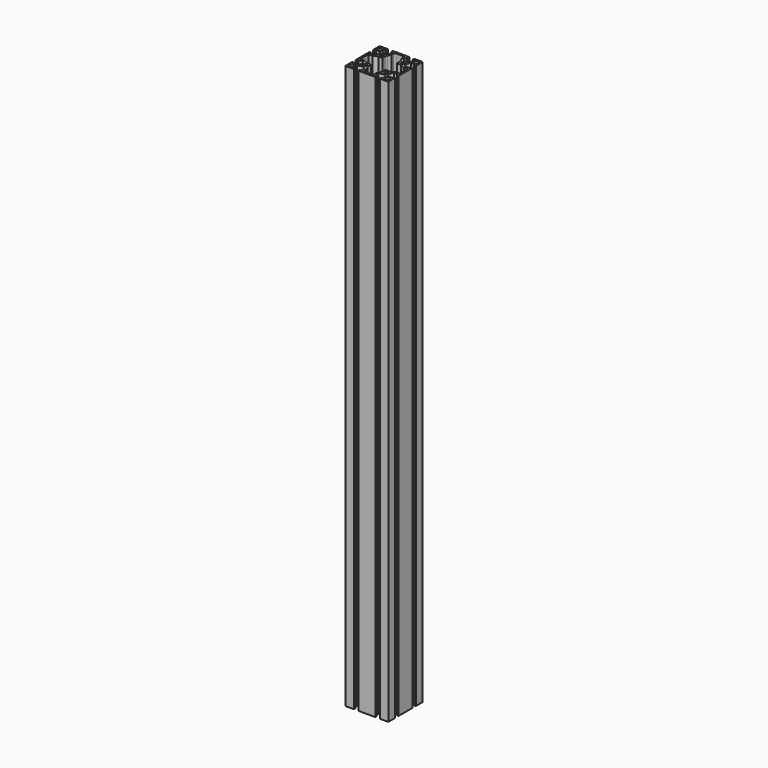
from build123d import *

# Parameters (mm, degrees)
F0_R     = 3
F0_R_2   = 2.5
F1_DEPTH = 787
F2_R     = 2
F3_R     = 7


# Not quite as in the source:
# - a feature names something its author has since deleted; it is built from what else it names


with BuildPart() as f1:
    # F0 (on Top) → F1 (new body)
    with BuildSketch(Plane.XY):
        with BuildLine():
            Line((18.15, -30), (30, -30))
            Line((30, -30), (30, -18.15))
            Line((30, -18.15), (27.5, -18.15))
            Line((27.5, -18.15), (27.5, -20.15))
            Line((27.5, -20.15), (21.5477069044, -20.15))
            ThreePointArc((21.5477069044, -20.15), (19.5, -15), (21.5477069044, -9.85))
            Line((21.5477069044, -9.85), (27.5, -9.85))
            Line((27.5, -9.85), (27.5, -11.85))
            Line((27.5, -11.85), (30, -11.85))
            Line((30, -11.85), (30, 11.85))
            Line((30, 11.85), (27.5, 11.85))
            Line((27.5, 11.85), (27.5, 9.85))
            Line((27.5, 9.85), (21.5477069044, 9.85))
            ThreePointArc((21.5477069044, 9.85), (19.5, 15), (21.5477069044, 20.15))
            Line((21.5477069044, 20.15), (27.5, 20.15))
            Line((27.5, 20.15), (27.5, 18.15))
            Line((27.5, 18.15), (30, 18.15))
            Line((30, 18.15), (30, 30))
            Line((30, 30), (18.15, 30))
            Line((18.15, 30), (18.15, 27.5))
            Line((18.15, 27.5), (20.15, 27.5))
            Line((20.15, 27.5), (20.15, 21.5477069044))
            ThreePointArc((20.15, 21.5477069044), (15, 19.5), (9.85, 21.5477069044))
            Line((9.85, 21.5477069044), (9.85, 27.5))
            Line((9.85, 27.5), (11.85, 27.5))
            Line((11.85, 27.5), (11.85, 30))
            Line((11.85, 30), (-11.85, 30))
            Line((-11.85, 30), (-11.85, 27.5))
            Line((-11.85, 27.5), (-9.85, 27.5))
            Line((-9.85, 27.5), (-9.85, 21.5477069044))
            ThreePointArc((-9.85, 21.5477069044), (-15, 19.5), (-20.15, 21.5477069044))
            Line((-20.15, 21.5477069044), (-20.15, 27.5))
            Line((-20.15, 27.5), (-18.15, 27.5))
            Line((-18.15, 27.5), (-18.15, 30))
            Line((-18.15, 30), (-30, 30))
            Line((-30, 30), (-30, 18.15))
            Line((-30, 18.15), (-27.5, 18.15))
            Line((-27.5, 18.15), (-27.5, 20.15))
            Line((-27.5, 20.15), (-21.5477069044, 20.15))
            ThreePointArc((-21.5477069044, 20.15), (-19.5, 15), (-21.5477069044, 9.85))
            Line((-21.5477069044, 9.85), (-27.5, 9.85))
            Line((-27.5, 9.85), (-27.5, 11.85))
            Line((-27.5, 11.85), (-30, 11.85))
            Line((-30, 11.85), (-30, -11.85))
            Line((-30, -11.85), (-27.5, -11.85))
            Line((-27.5, -11.85), (-27.5, -9.85))
            Line((-27.5, -9.85), (-21.5477069044, -9.85))
            ThreePointArc((-21.5477069044, -9.85), (-19.5, -15), (-21.5477069044, -20.15))
            Line((-21.5477069044, -20.15), (-27.5, -20.15))
            Line((-27.5, -20.15), (-27.5, -18.15))
            Line((-27.5, -18.15), (-30, -18.15))
            Line((-30, -18.15), (-30, -30))
            Line((-30, -30), (-18.15, -30))
            Line((-18.15, -30), (-18.15, -27.5))
            Line((-18.15, -27.5), (-20.15, -27.5))
            Line((-20.15, -27.5), (-20.15, -21.5477069044))
            ThreePointArc((-20.15, -21.5477069044), (-15, -19.5), (-9.85, -21.5477069044))
            Line((-9.85, -21.5477069044), (-9.85, -27.5))
            Line((-9.85, -27.5), (-11.85, -27.5))
            Line((-11.85, -27.5), (-11.85, -30))
            Line((-11.85, -30), (11.85, -30))
            Line((11.85, -30), (11.85, -27.5))
            Line((11.85, -27.5), (9.85, -27.5))
            Line((9.85, -27.5), (9.85, -21.5477069044))
            ThreePointArc((9.85, -21.5477069044), (15, -19.5), (20.15, -21.5477069044))
            Line((20.15, -21.5477069044), (20.15, -27.5))
            Line((20.15, -27.5), (18.15, -27.5))
            Line((18.15, -27.5), (18.15, -30))
        make_face()
        with Locations((-25, -25)):
            Circle(F0_R, mode=Mode.SUBTRACT)
        with Locations((-15, -15)):
            Circle(F0_R_2, mode=Mode.SUBTRACT)
        with Locations((25, -25)):
            Circle(F0_R, mode=Mode.SUBTRACT)
        with Locations((15, -15)):
            Circle(F0_R_2, mode=Mode.SUBTRACT)
        with Locations((-25, 25)):
            Circle(F0_R, mode=Mode.SUBTRACT)
        with Locations((-15, 15)):
            Circle(F0_R_2, mode=Mode.SUBTRACT)
        Polygon((-7, 22), (-7, 27.5), (0, 27.5), (7, 27.5), (7, 22), (10, 16), (10, 10), (16, 10), (22, 7), (27.5, 7), (27.5, 0), (27.5, -7), (22, -7), (16, -10), (10, -10), (10, -16), (7, -22), (7, -27.5), (0, -27.5), (-7, -27.5), (-7, -22), (-10, -16), (-10, -10), (-16, -10), (-22, -7), (-27.5, -7), (-27.5, 0), (-27.5, 7), (-22, 7), (-16, 10), (-10, 10), (-10, 16), align=None, mode=Mode.SUBTRACT)
        with Locations((15, 15)):
            Circle(F0_R_2, mode=Mode.SUBTRACT)
        with Locations((25, 25)):
            Circle(F0_R, mode=Mode.SUBTRACT)
    extrude(amount=F1_DEPTH)

    # F2
    f2_edges = [f1.edges().sort_by_distance(p)[0] for p in [
        (-7, 27.5, 393.5),
        (7, 27.5, 393.5),
    ]]
    fillet(f2_edges, radius=F2_R)

    # F3
    f3_edges = [f1.edges().sort_by_distance(p)[0] for p in [
        (-10, 16, 393.5),
        (10, 16, 393.5),
    ]]
    fillet(f3_edges, radius=F3_R)


solid = f1.part
